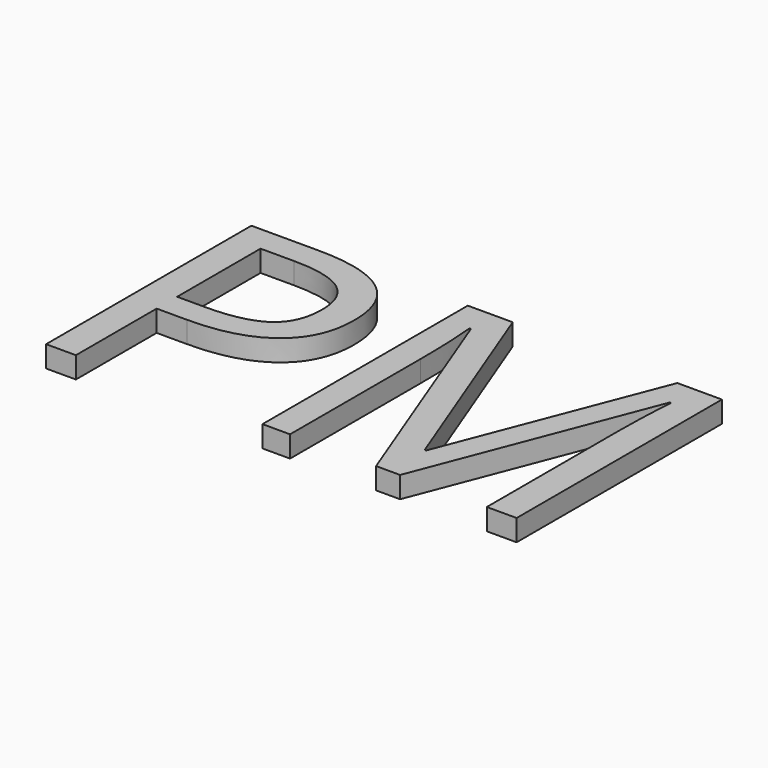
from build123d import *

# Parameters (mm, degrees)
F0_TEXT_SIZE = 33.5738062859
F1_DEPTH     = 2


# Not quite as in the source:
# - Text() gives the source's letters only with a copy of the font that has no kerning and outlines rounded to 1/6400 em; it was checked with that copy


with BuildPart() as f1:
    # F0 (on Top) → F1 (new body)
    with BuildSketch(Plane.XY):
        with Locations((-43.1545525789, -69.2813917994)):
            Text('PM', F0_TEXT_SIZE, font='Open Sans', text_align=(TextAlign.LEFT, TextAlign.BOTTOM))
    extrude(amount=F1_DEPTH)


solid = f1.part
